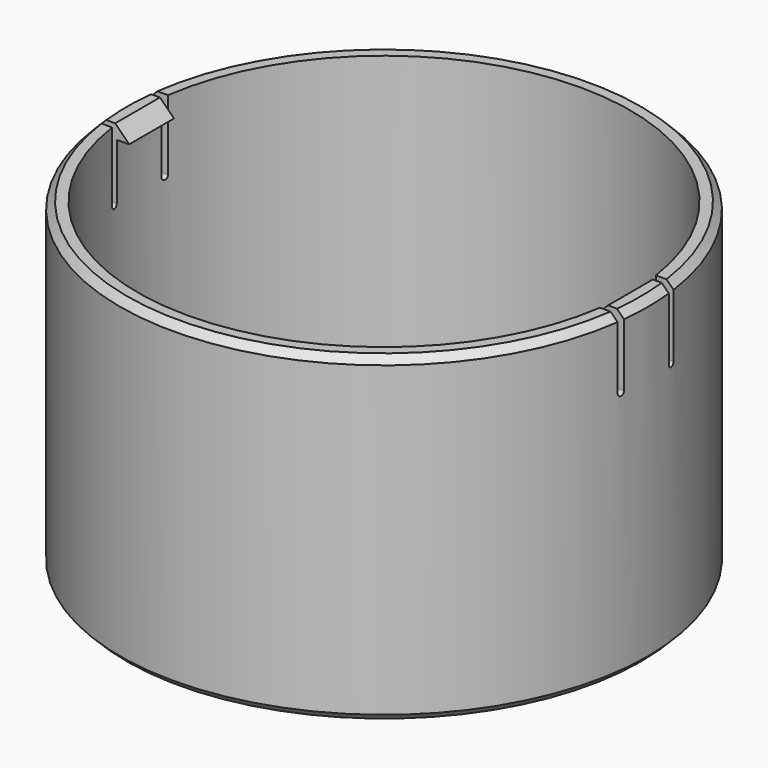
from build123d import *

# Parameters (mm, degrees)
F0_R          = 18.875
F0_R_2        = 17.625
F1_DEPTH      = 23
F0_R_3        = 16
F2_DEPTH      = 1
F3_SIZE       = 0.5
F5_DEPTH      = 25
F5_DEPTH_BACK = 25
F7_DEPTH      = 1
F8_SIZE       = 0.99999


# Not quite as in the source:
# - a fillet or chamfer is up to 0.001 mm smaller than in the source, because OpenCascade refuses the exact size


with BuildPart() as f1:
    # F0 (on Top) → F1 (new body)
    with BuildSketch(Plane.XY):
        Circle(F0_R)
        Circle(F0_R_2, mode=Mode.SUBTRACT)
    extrude(amount=F1_DEPTH)

    # F0 (on Top) → F2 (join)
    with BuildSketch(Plane.XY):
        Circle(F0_R_2)
        Circle(F0_R_3, mode=Mode.SUBTRACT)
    extrude(amount=F2_DEPTH)

    # F3
    f3_edges = [f1.edges().sort_by_distance(p)[0] for p in [
        (-18.875, 0, 0),
        (-16, 0, 0),
        (-18.875, 0, 23),
    ]]
    chamfer(f3_edges, length=F3_SIZE)

    # F4 (on Right) → F5 (cut, two sides)
    with BuildSketch(Plane.YZ) as f5_sk:
        with BuildLine():
            Line((-2.5, 18), (-2, 18))
            ThreePointArc((-2, 18), (-2.25, 18.25), (-2.5, 18))
        make_face()
        with BuildLine():
            ThreePointArc((-2.5, 18), (-2.25, 17.75), (-2, 18))
            Line((-2, 18), (-2.5, 18))
        make_face()
        with BuildLine():
            ThreePointArc((-2.5, 18), (-2.25, 18.25), (-2, 18))
            Line((-2, 18), (-2, 23))
            Line((-2, 23), (-2.5, 23))
            Line((-2.5, 23), (-2.5, 18))
        make_face()
        with BuildLine():
            Line((2.5, 23), (2, 23))
            Line((2, 23), (2, 18))
            ThreePointArc((2, 18), (2.25, 18.25), (2.5, 18))
            Line((2.5, 18), (2.5, 23))
        make_face()
        with BuildLine():
            ThreePointArc((2.5, 18), (2.25, 18.25), (2, 18))
            Line((2, 18), (2.5, 18))
        make_face()
        with BuildLine():
            Line((2.5, 18), (2, 18))
            ThreePointArc((2, 18), (2.25, 17.75), (2.5, 18))
        make_face()
    extrude(amount=-F5_DEPTH, mode=Mode.SUBTRACT)
    extrude(f5_sk.sketch, amount=F5_DEPTH_BACK, mode=Mode.SUBTRACT)

    # F6 (on face) → F7 (join)
    with BuildSketch(Plane.XY.offset(23)):
        with BuildLine():
            ThreePointArc((-17.5111571577, 2), (-17.5965162732, 1.001618714), (-17.625, 0))
            Line((-17.625, 0), (-16.625, 0))
            Line((-16.625, 0), (-16.625, 2))
            Line((-16.625, 2), (-17.5111571577, 2))
        make_face()
        with BuildLine():
            Line((-16.625, 0), (-17.625, 0))
            ThreePointArc((-17.625, 0), (-17.5965162732, -1.001618714), (-17.5111571577, -2))
            Line((-17.5111571577, -2), (-16.625, -2))
            Line((-16.625, -2), (-16.625, 0))
        make_face()
        Polygon((17.8884946657, 2), (17.5111571577, 2), (16.625, 2), (16.625, 0), (16.625, -2), (17.8884946657, -2), align=None)
    extrude(amount=-F7_DEPTH)

    # F8 (size 1 in the source; OpenCascade refuses exactly that, so slightly less here)
    f8_edges = [f1.edges().sort_by_distance(p)[0] for p in [
        (-16.625, 0, 23),
        (16.625, 0, 23),
    ]]
    chamfer(f8_edges, length=F8_SIZE)


solid = f1.part
